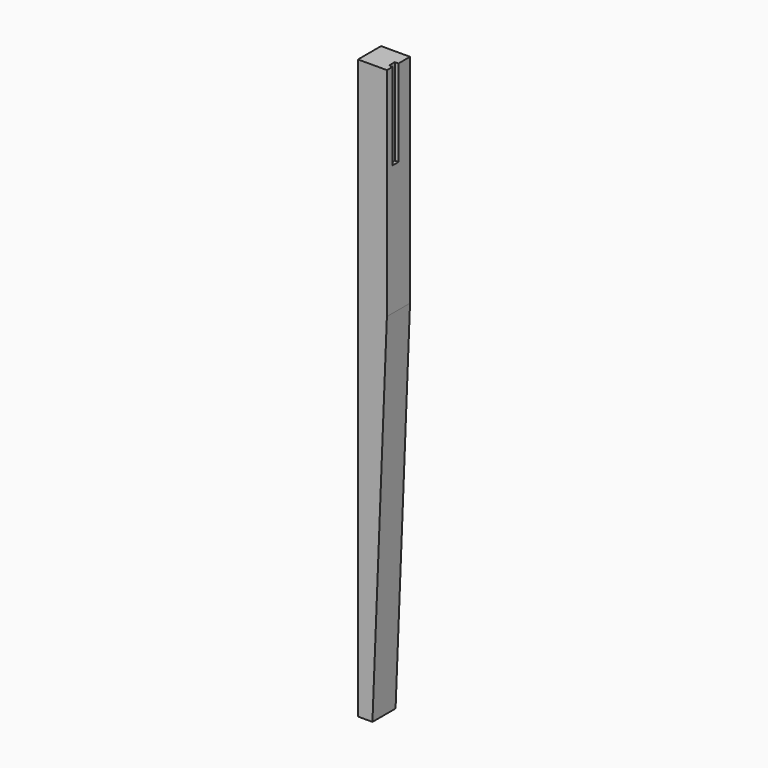
from build123d import *

# Parameters (mm, degrees)
F1_DEPTH = 50.8
F2_W     = 12.7
F2_H     = 152.4
F3_DEPTH = 6.35


# Not quite as in the source:
# - a feature names something its author has since deleted; it is built from what else it names


with BuildPart() as f1:
    # F0 (on Front) → F1 (new body)
    with BuildSketch(Plane.XZ):
        Polygon((50.8, 0), (0, 0), (0, -1016), (25.4, -1016), (50.8, -381), align=None)
    extrude(amount=-F1_DEPTH)

    # F2 (on face) → F3 (cut)
    with BuildSketch(Plane.YZ.offset(50.8)):
        with Locations((19.05, -76.2)):
            Rectangle(F2_W, F2_H)
    extrude(amount=-F3_DEPTH, mode=Mode.SUBTRACT)


solid = f1.part
